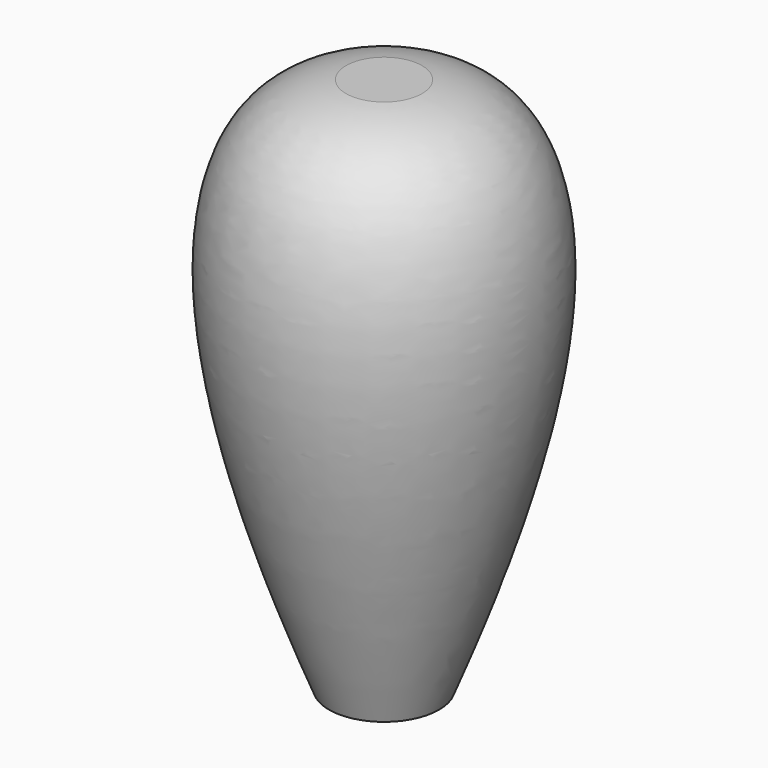
from build123d import *


# Not quite as in the source:
# - ends of sketch curves that miss each other by under 0.0002 mm in the source are joined


with BuildPart() as f1:
    # F0 (on Front) → F1 (revolve)
    with BuildSketch(Plane.XZ):
        with BuildLine():
            Line((0, 44.8796040858), (0, 25.4983261479))
            Line((0, 25.4983261479), (1.5, 25.4983261479))
            ThreePointArc((1.5, 25.4983261479), (2.7242544852, 24.3306639644), (3.175, 22.7000007558))
            Line((3.175, 22.7000007558), (3.175, 0))
            Line((3.175, 0), (4.6101, 7.558e-07))
            add(Edge.make_bspline(
                [(3.175, 44.8796040858), (8.1088727658, 44.2273590028), (15.427827503, 35.7047061614), (11.1691896678, 16.3609262944), (4.6101, 7.558e-07)],
                knots=[0.0617585703, 0.0617585703, 0.0617585703, 0.0617585703, 0.3785360097, 1, 1, 1, 1], degree=3))
            Line((3.175, 44.8796040858), (0, 44.8796040858))
        make_face()
    revolve(axis=Axis((0, 0, 33.8500003779), (0, 0, 1)))


solid = f1.part
